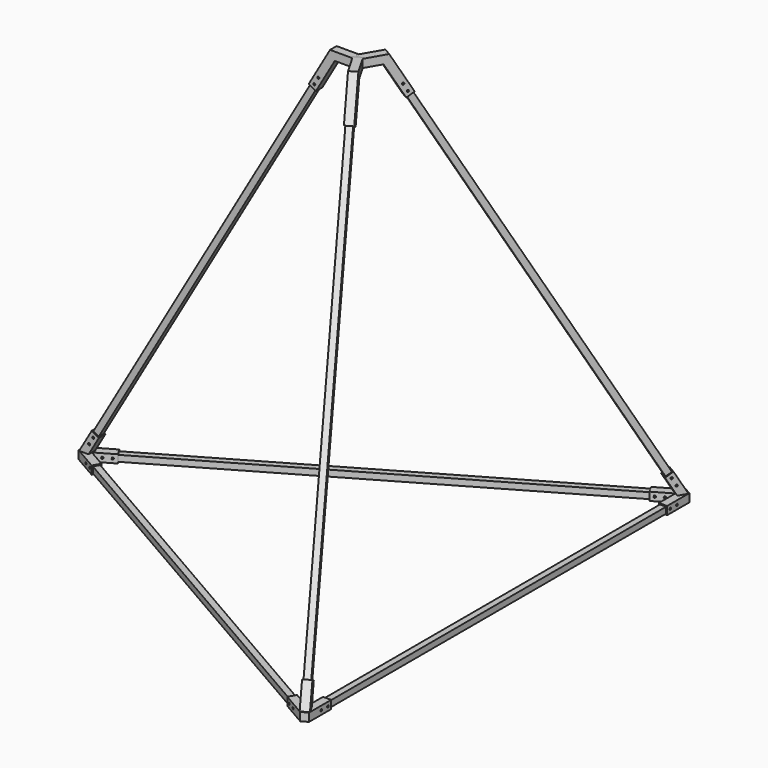
from build123d import *

# Parameters (mm, degrees)
F1_DEPTH       = 50.8
F5_DEPTH       = 25.4
F7_W           = 38.1
F7_H           = 38.1
F10_DEPTH      = 101.6
F8_W           = 38.1
F8_H           = 38.1
F11_DEPTH      = 101.6
F9_W           = 38.1
F9_H           = 38.1
F12_DEPTH      = 101.6
F13_W          = 38.1
F13_H          = 38.1
F14_DEPTH      = 101.6
F15_DEPTH      = 2794
F17_DEPTH      = 25.4
F20_DEPTH      = 6.35
F21_DEPTH      = 6.35
F22_R          = 6.35
F26_DEPTH      = 50.8
F23_R          = 6.35
F27_DEPTH      = 50.8
F24_R          = 6.35
F28_DEPTH      = 50.8
F25_R          = 6.35
F29_DEPTH      = 50.8
F30_COUNT      = 3
F31_W          = 38.1
F31_H          = 38.1
F32_DEPTH      = 101.6
F32_DEPTH_BACK = 2707.2158832962
F33_W          = 38.1
F33_H          = 38.1
F34_DEPTH      = 101.6
F34_DEPTH_BACK = 2707.2158832962
F35_W          = 38.1
F35_H          = 38.1
F36_DEPTH      = 101.6
F36_DEPTH_BACK = 2707.2158832962


with BuildPart() as f1:
    # F0 (on Top) → F1 (new body)
    with BuildSketch(Plane.XY):
        Polygon((-1541.0147737194, -63.5), (-1651, 0), (-1541.0147737194, 63.5), (-1566.4147737194, 107.4940905122), (-1715.0628941156, 21.6720581869), (-1715.0628941156, -21.6720581869), (-1566.4147737194, -107.4940905122), align=None)
    extrude(amount=F1_DEPTH)

    # F4 (on line) → F5 (join, symmetric)
    with BuildSketch(Plane.XZ):
        Polygon((-1651, 50.8), (-1587.5, 160.7852262806), (-1631.4940905123, 186.1852262806), (-1709.6587873497, 50.8), align=None)
    extrude(amount=F5_DEPTH, both=True)

    # F7 (on face) → F10 (cut)
    with BuildSketch(Plane(origin=(-1128.2647737194, 651.4039708241, 0), x_dir=(0.5, 0.8660254038, 0), z_dir=(0.8660254038, -0.5, 0))):
        with Locations((-850.9, 25.4)):
            Rectangle(F7_W, F7_H)
    extrude(amount=-F10_DEPTH, mode=Mode.SUBTRACT)

    # F8 (on face) → F11 (cut)
    with BuildSketch(Plane(origin=(-1128.2647737194, -651.4039708241, 0), x_dir=(-0.5, 0.8660254038, 0), z_dir=(0.8660254038, 0.5, 0))):
        with Locations((850.9, 25.4)):
            Rectangle(F8_W, F8_H)
    extrude(amount=-F11_DEPTH, mode=Mode.SUBTRACT)

    # F9 (on face) → F12 (cut)
    with BuildSketch(Plane(origin=(-327.2529547439, 0, -566.8187445434), x_dir=(0.8660254038, 0, -0.5), z_dir=(0.5, 0, 0.8660254038))):
        with Locations((-1480.6079416481, 0)):
            Rectangle(F9_W, F9_H)
    extrude(amount=-F12_DEPTH, mode=Mode.SUBTRACT)

    # F22 (on face) → F26 (cut, through all)
    with BuildSketch(Plane.XZ.offset(25.4)):
        with Locations((-1622.1970452561, 151.4881810245)):
            Circle(F22_R)
        with Locations((-1647.5970452561, 107.4940905123)):
            Circle(F22_R)
    extrude(amount=-F26_DEPTH, mode=Mode.SUBTRACT)

    # F23 (on face) → F27 (cut, through all)
    with BuildSketch(Plane(origin=(-438.15, -758.8980613363, 0), x_dir=(0.8660254038, -0.5, 0), z_dir=(-0.5, -0.8660254038, 0))):
        with Locations((-1328.2079416481, 25.4)):
            Circle(F23_R)
        with Locations((-1379.0079416481, 25.4)):
            Circle(F23_R)
    extrude(amount=-F27_DEPTH, mode=Mode.SUBTRACT)

    # F24 (on face) → F28 (cut, through all)
    with BuildSketch(Plane(origin=(-438.15, 758.8980613363, 0), x_dir=(-0.8660254038, -0.5, 0), z_dir=(-0.5, 0.8660254038, 0))):
        with Locations((1328.2079416481, 25.4)):
            Circle(F24_R)
        with Locations((1379.0079416481, 25.4)):
            Circle(F24_R)
    extrude(amount=-F28_DEPTH, mode=Mode.SUBTRACT)


with BuildPart() as f14:
    # F13 (on face) → F14 (new body)
    with BuildSketch(Plane(origin=(-327.2529547439, 0, -566.8187445434), x_dir=(0.8660254038, 0, -0.5), z_dir=(0.5, 0, 0.8660254038))):
        with Locations((-1480.6079416481, 0)):
            Rectangle(F13_W, F13_H)
    extrude(amount=-F14_DEPTH)

    # F15 (add): a face of the model
    f15_faces = [f14.faces().sort_by_distance(p)[0] for p in [
        (-1609.4970452561, 0, 173.4852262806),
    ]]
    extrude(f15_faces, amount=F15_DEPTH)


with BuildPart() as f17:
    # F16 (on line) → F17 (new body, symmetric)
    with BuildSketch(Plane.XZ):
        Polygon((-285.2940905123, 2517.8720234298), (-279.7948291982, 2514.6970234298), (-228.9948291982, 2602.6852044543), (-195.999261314, 2583.6352044543), (-246.799261314, 2495.6470234298), (-241.3, 2492.4720234298), (-123.4245187336, 2696.63834595), (0, 2696.63834595), (0, 2747.43834595), (-152.7539124084, 2747.43834595), align=None)
    extrude(amount=F17_DEPTH, both=True)

    # F18 (on face) → F20 (join)
    with BuildSketch(Plane.XZ.offset(25.4)):
        Polygon((-195.999261314, 2583.6352044543), (-228.9948291982, 2602.6852044543), (-279.7948291982, 2514.6970234298), (-246.799261314, 2495.6470234298), align=None)
    extrude(amount=-F20_DEPTH)

    # F19 (on face) → F21 (join)
    with BuildSketch(Plane(origin=(0, 25.4, 0), x_dir=(-1, 0, 0), z_dir=(0, 1, 0))):
        Polygon((279.7948291982, 2514.6970234298), (228.9948291982, 2602.6852044543), (195.999261314, 2583.6352044543), (246.799261314, 2495.6470234298), align=None)
    extrude(amount=-F21_DEPTH)

    # F25 (on face) → F29 (cut, through all)
    with BuildSketch(Plane.XZ.offset(25.4)):
        with Locations((-250.5970452561, 2527.169068686)):
            Circle(F25_R)
        with Locations((-225.1970452561, 2571.1631591982)):
            Circle(F25_R)
    extrude(amount=-F29_DEPTH, mode=Mode.SUBTRACT)


with BuildPart() as f30_1:
    # F30: instance of F1
    add(f1.part.rotate(Axis((0, 0, -7.7725015581), (0, 0, -1)), 1 * 360 / F30_COUNT))


with BuildPart() as f30_2:
    # F30: instance of F1
    add(f1.part.rotate(Axis((0, 0, -7.7725015581), (0, 0, -1)), 2 * 360 / F30_COUNT))


with BuildPart() as f30_3:
    # F30: instance of F14
    add(f14.part.rotate(Axis((0, 0, -7.7725015581), (0, 0, -1)), 1 * 360 / F30_COUNT))


with BuildPart() as f30_4:
    # F30: instance of F14
    add(f14.part.rotate(Axis((0, 0, -7.7725015581), (0, 0, -1)), 2 * 360 / F30_COUNT))


with BuildPart() as f30_5:
    # F30: instance of F17
    add(f17.part.rotate(Axis((0, 0, -7.7725015581), (0, 0, -1)), 1 * 360 / F30_COUNT))


with BuildPart() as f30_6:
    # F30: instance of F17
    add(f17.part.rotate(Axis((0, 0, -7.7725015581), (0, 0, -1)), 2 * 360 / F30_COUNT))


with BuildPart() as f32:
    # F31 (on face) → F32 (new body, two sides)
    with BuildSketch(Plane(origin=(-1128.2647737194, 651.4039708241, 0), x_dir=(0.5, 0.8660254038, 0), z_dir=(0.8660254038, -0.5, 0))) as f32_sk:
        with Locations((-850.9, 25.4)):
            Rectangle(F31_W, F31_H)
    extrude(amount=-F32_DEPTH)
    extrude(f32_sk.sketch, amount=F32_DEPTH_BACK)


with BuildPart() as f34:
    # F33 (on face) → F34 (new body, two sides)
    with BuildSketch(Plane(origin=(-1128.2647737194, -651.4039708241, 0), x_dir=(-0.5, 0.8660254038, 0), z_dir=(0.8660254038, 0.5, 0))) as f34_sk:
        with Locations((850.9, 25.4)):
            Rectangle(F33_W, F33_H)
    extrude(amount=-F34_DEPTH)
    extrude(f34_sk.sketch, amount=F34_DEPTH_BACK)


with BuildPart() as f36:
    # F35 (on face) → F36 (new body, two sides)
    with BuildSketch(Plane(origin=(0, -1302.8079416481, 0), x_dir=(-1, 0, 0), z_dir=(0, 1, 0))) as f36_sk:
        with Locations((-850.9, 25.4)):
            Rectangle(F35_W, F35_H)
    extrude(amount=-F36_DEPTH)
    extrude(f36_sk.sketch, amount=F36_DEPTH_BACK)


solid = Compound([f1.part, f14.part, f17.part, f30_1.part, f30_2.part, f30_3.part, f30_4.part, f30_5.part, f30_6.part, f32.part, f34.part, f36.part])
